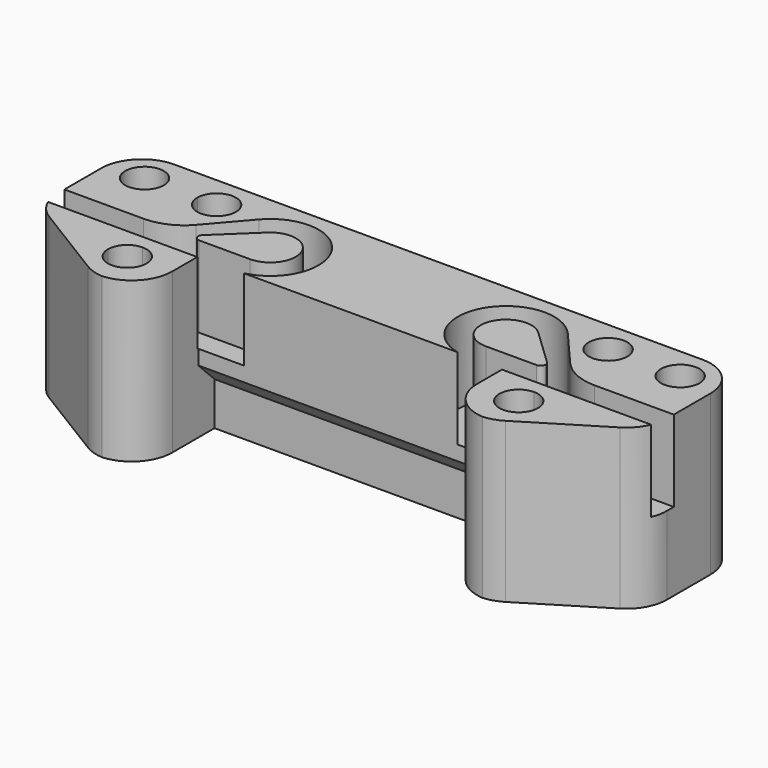
from build123d import *

# Parameters (mm, degrees)
F1_DEPTH    = 15.7
F2_W        = 10.0960650777
F2_H        = 2.4
F3_DEPTH    = 8
F4_R        = 5
F5_T1_DEPTH = 26.8923143391
F5_T3_DEPTH = 21.3473434867
F5_T5_DEPTH = 35.7
F6_W        = 15
F6_H        = 6.25
F7_DEPTH    = 2
F8_SIZE     = 1.99999


# Not quite as in the source:
# - a fillet or chamfer that OpenCascade refuses, or shapes differently, is made with other operations: its cross-section is extruded or revolved along the edge and cut away or added
# - a fillet or chamfer is up to 0.001 mm smaller than in the source, because OpenCascade refuses the exact size


with BuildPart() as f1:
    # F0 (on Top) → F1 (new body)
    with BuildSketch(Plane.XY):
        Polygon((30, 9), (0, 9), (0, -1.8), (15, -1.8), (15, -9), (19.5954625243, -9), (30, -2.6151265483), align=None)
        with BuildLine():
            ThreePointArc((21.17, -5.2), (17.9264971157, -6.5435028843), (19.27, -3.3))
            ThreePointArc((19.27, -3.3), (20.6135028843, -3.8564971157), (21.17, -5.2))
        make_face(mode=Mode.SUBTRACT)
        with BuildLine():
            ThreePointArc((19.27, 3.9), (17.9264971157, 7.1435028843), (21.17, 5.8))
            ThreePointArc((21.17, 5.8), (20.6135028843, 4.4564971157), (19.27, 3.9))
        make_face(mode=Mode.SUBTRACT)
        with BuildLine():
            ThreePointArc((24.47, 5.8), (26.37, 7.7), (28.27, 5.8))
            ThreePointArc((28.27, 5.8), (26.37, 3.9), (24.47, 5.8))
        make_face(mode=Mode.SUBTRACT)
    extrude(amount=F1_DEPTH)

    # F2 (on face) → F3 (cut)
    with BuildSketch(Plane.XY.offset(15.7)):
        with BuildLine():
            ThreePointArc((11.6039349223, 0.3250306588), (9.2827431951, 3.7535073497), (13.3280728534, 4.6353754864))
            Line((13.3280728534, 4.6353754864), (16.2527744297, 1.8499454137))
            ThreePointArc((16.2527744297, 1.8499454137), (16.328577113, 2.3348713274), (16.3539349223, 2.8250306588))
            ThreePointArc((16.3539349223, 2.8250306588), (16.0563093355, 4.479981439), (15.200729834, 5.9275403467))
            ThreePointArc((15.200729834, 5.9275403467), (7.5407755063, 5.2853630672), (10.5215341623, -1.8))
            Line((10.5215341623, -1.8), (12.6863356823, -1.8))
            ThreePointArc((12.6863356823, -1.8), (14.376262754, -1.0320016711), (15.6428085277, 0.3250306588))
            Line((15.6428085277, 0.3250306588), (11.6039349223, 0.3250306588))
        make_face()
        with BuildLine():
            ThreePointArc((16.3539349223, 2.8250306588), (16.328577113, 2.3348713274), (16.2527744297, 1.8499454137))
            Line((16.2527744297, 1.8499454137), (16.9487625085, 1.1870996243))
            ThreePointArc((16.9487625085, 1.1870996243), (17.0635074373, 1.0219903081), (17.1039349223, 0.8250306588))
            ThreePointArc((17.1039349223, 0.8250306588), (16.9574883129, 0.4714772682), (16.6039349223, 0.3250306588))
            Line((16.6039349223, 0.3250306588), (15.6428085277, 0.3250306588))
            ThreePointArc((15.6428085277, 0.3250306588), (14.376262754, -1.0320016711), (12.6863356823, -1.8))
            Line((12.6863356823, -1.8), (15, -1.8))
            Line((15, -1.8), (15, -1.9249693412))
            Line((15, -1.9249693412), (19.9039349223, -1.9249693412))
            Line((19.9039349223, -1.9249693412), (19.9039349223, 0.4750306588))
            Line((19.9039349223, 0.4750306588), (15.200729834, 5.9275403467))
            ThreePointArc((15.200729834, 5.9275403467), (16.0563093355, 4.479981439), (16.3539349223, 2.8250306588))
        make_face()
        with Locations((24.9519674612, -0.7249693412)):
            Rectangle(F2_W, F2_H)
    extrude(amount=-F3_DEPTH, mode=Mode.SUBTRACT)

    # F4
    f4_edges = [f1.edges().sort_by_distance(p)[0] for p in [
        (19.903935, 0.475031, 11.7),
    ]]
    fillet(f4_edges, radius=F4_R)

    # F5: fillet of radius 4 on 4 edges, made by hand

    # F5_s2 → F5_t1 (cut)
    with BuildSketch(Plane.XY.offset(-5.5961571696)):
        with BuildLine():
            ThreePointArc((30, -0.3766636805), (29.4905957559, -2.3300559271), (28.0921293656, -3.7859150232))
            Line((28.0921293656, -3.7859150232), (30, -2.6151265483))
            Line((30, -2.6151265483), (30, -0.3766636805))
        make_face()
    extrude(amount=F5_T1_DEPTH, mode=Mode.SUBTRACT)

    # F5_s4 → F5_t3 (cut)
    with BuildSketch(Plane.XY.offset(-2.8236717433)):
        with BuildLine():
            ThreePointArc((20.5581231925, -8.4092513427), (19.5529608525, -8.8494808332), (18.465993827, -9))
            Line((18.465993827, -9), (19.5954625243, -9))
            Line((19.5954625243, -9), (20.5581231925, -8.4092513427))
        make_face()
    extrude(amount=F5_T3_DEPTH, mode=Mode.SUBTRACT)

    # F5_s6 → F5_t5 (cut)
    with BuildSketch(Plane.XY.offset(-10)):
        with BuildLine():
            ThreePointArc((15, -5), (16.1715728753, -7.8284271247), (19, -9))
            Line((19, -9), (15, -9))
            Line((15, -9), (15, -5))
        make_face()
        with BuildLine():
            ThreePointArc((30, 5), (28.8284271247, 7.8284271247), (26, 9))
            Line((26, 9), (30, 9))
            Line((30, 9), (30, 5))
        make_face()
    extrude(amount=F5_T5_DEPTH, mode=Mode.SUBTRACT)

    # F6 (on face) → F7 (cut)
    with BuildSketch(Plane.XZ.offset(1.8)):
        with Locations((7.5, 3.125)):
            Rectangle(F6_W, F6_H)
    extrude(amount=-F7_DEPTH, mode=Mode.SUBTRACT)

    # F8 (size 2 in the source; OpenCascade refuses exactly that, so slightly less here)
    f8_edges = [f1.edges().sort_by_distance(p)[0] for p in [
        (7.5, 0.2, 6.25),
    ]]
    chamfer(f8_edges, length=F8_SIZE)

    # F9: F1 across plane


with BuildPart() as f1_1:
    add(f1.part)
    add(f1.part.mirror(Plane.YZ))


solid = f1_1.part
